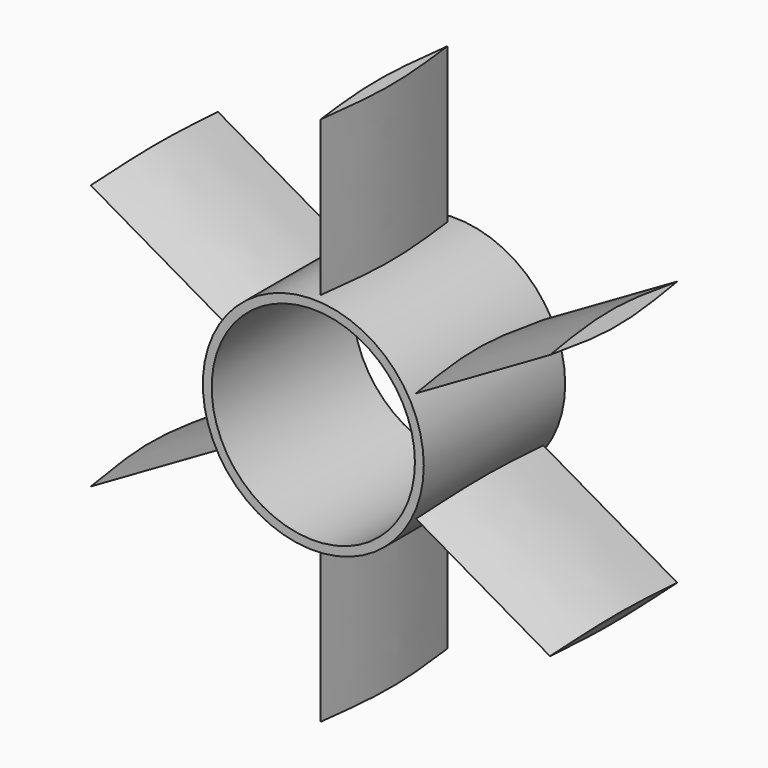
from build123d import *

# Parameters (mm, degrees)
F0_R            = 15.875
F0_R_2          = 14.605
F1_DEPTH        = 25.4
F4_DEPTH        = 22.225
F4_COPIES_COUNT = 6


# Not quite as in the source:
# - a length typed as a fraction of an inch, garbled in the dataset ("3 / 203.2 mm" for 3/8 in), is restored
# - a pattern or mirror of a feature is missing from the dataset's text; its kind, count and spacing are read off the source's solid


with BuildPart() as f1:
    # F0 (on Front) → F1 (new body)
    with BuildSketch(Plane.XZ):
        Circle(F0_R)
        Circle(F0_R_2, mode=Mode.SUBTRACT)
    extrude(amount=F1_DEPTH)


with BuildPart() as f4:
    # F3 (on offset) → F4 (new body)
    with BuildSketch(Plane.XY.offset(15.875)):
        with BuildLine():
            add(Edge.make_bspline(
                [(0, -1.27), (-0.47625, -5.08), (-0.9525, -8.89), (-0.9525, -12.7)],
                knots=[0, 0, 0, 0, 0.5, 0.5, 0.5, 0.5], degree=3))
            Line((-0.9525, -12.7), (0.9525, -12.7))
            add(Edge.make_bspline(
                [(0, -1.27), (0.47625, -5.08), (0.9525, -8.89), (0.9525, -12.7)],
                knots=[0, 0, 0, 0, 0.5, 0.5, 0.5, 0.5], degree=3))
        make_face()
        with BuildLine():
            Line((0.9525, -12.7), (-0.9525, -12.7))
            add(Edge.make_bspline(
                [(-0.9525, -12.7), (-0.9525, -16.51), (-0.47625, -20.32), (0, -24.13)],
                knots=[0.5, 0.5, 0.5, 0.5, 1, 1, 1, 1], degree=3))
            add(Edge.make_bspline(
                [(0.9525, -12.7), (0.9525, -16.51), (0.47625, -20.32), (0, -24.13)],
                knots=[0.5, 0.5, 0.5, 0.5, 1, 1, 1, 1], degree=3))
        make_face()
    extrude(amount=F4_DEPTH)


with BuildPart() as f4_copies_1:
    # F4_copies: instance of F4
    add(f4.part.rotate(Axis((0, 0, 0), (0, 1, 0)), 1 * 360 / F4_COPIES_COUNT))


with BuildPart() as f4_copies_2:
    # F4_copies: instance of F4
    add(f4.part.rotate(Axis((0, 0, 0), (0, 1, 0)), 2 * 360 / F4_COPIES_COUNT))


with BuildPart() as f4_copies_3:
    # F4_copies: instance of F4
    add(f4.part.rotate(Axis((0, 0, 0), (0, 1, 0)), 3 * 360 / F4_COPIES_COUNT))


with BuildPart() as f4_copies_4:
    # F4_copies: instance of F4
    add(f4.part.rotate(Axis((0, 0, 0), (0, 1, 0)), 4 * 360 / F4_COPIES_COUNT))


with BuildPart() as f4_copies_5:
    # F4_copies: instance of F4
    add(f4.part.rotate(Axis((0, 0, 0), (0, 1, 0)), 5 * 360 / F4_COPIES_COUNT))


solid = Compound([f1.part, f4.part, f4_copies_1.part, f4_copies_2.part, f4_copies_3.part, f4_copies_4.part, f4_copies_5.part])
